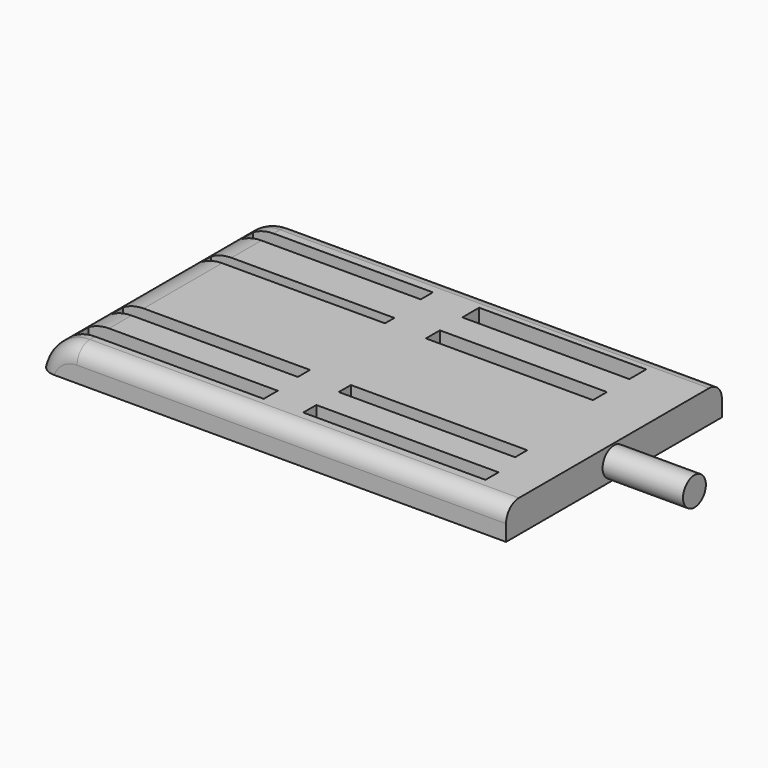
from build123d import *

# Parameters (mm, degrees)
F0_W        = 147.8525847197
F0_H        = 85.1719379425
F0_W_2      = 59.7309665754
F0_H_2      = 5.5306423455
F0_W_3      = 58.9935472235
F0_H_3      = 4.7932267189
F0_W_4      = 57.5187108479
F0_H_4      = 5.1619354635
F0_W_5      = 55.6751615368
F0_W_6      = 57.8874191269
F0_H_5      = 3.6870967597
F0_W_7      = 56.7812863737
F0_H_6      = 4.7932248563
F0_W_8      = 52.7254838962
F0_H_7      = 5.5306442082
F0_H_8      = 6.6367760301
F1_DEPTH    = 10.16
F2_T1_DEPTH = 147.3889774092
F3_R        = 5.08
F4_R        = 4.5031383634
F5_DEPTH    = 25.4


# Not quite as in the source:
# - a fillet or chamfer that OpenCascade refuses, or shapes differently, is made with other operations: its cross-section is extruded or revolved along the edge and cut away or added


with BuildPart() as f1:
    # F0 (on Top) → F1 (new body)
    with BuildSketch(Plane.XY):
        Rectangle(F0_W, F0_H)
        with Locations((-38.0981913768, -32.7256983146)):
            Rectangle(F0_W_2, F0_H_2, mode=Mode.SUBTRACT)
        with Locations((-38.4669010527, -18.7147296965)):
            Rectangle(F0_W_3, F0_H_3, mode=Mode.SUBTRACT)
        with Locations((32.6940652449, -32.5413448736)):
            Rectangle(F0_W_4, F0_H_4, mode=Mode.SUBTRACT)
        with Locations((31.7722905893, -18.7147296965)):
            Rectangle(F0_W_5, F0_H_3, mode=Mode.SUBTRACT)
        with Locations((-39.019965101, 16.4970448241)):
            Rectangle(F0_W_6, F0_H_5, mode=Mode.SUBTRACT)
        with Locations((-39.5730314776, 32.535915263)):
            Rectangle(F0_W_7, F0_H_6, mode=Mode.SUBTRACT)
        with Locations((29.1913239053, 17.4188185483)):
            Rectangle(F0_W_8, F0_H_7, mode=Mode.SUBTRACT)
        with Locations((29.1913239053, 32.3515608907)):
            Rectangle(F0_W_8, F0_H_8, mode=Mode.SUBTRACT)
    extrude(amount=F1_DEPTH)

    # F2: fillet of radius 12.7 on 1 edges, made by hand

    # F2_s2 → F2_t1 (cut)
    with BuildSketch(Plane.XZ.offset(-73.6944887046)):
        with BuildLine():
            ThreePointArc((-73.9262923598, 0), (-69.5150697233, 7.2973776994), (-61.4828844665, 10.16))
            Line((-61.4828844665, 10.16), (-73.9262923598, 10.16))
            Line((-73.9262923598, 10.16), (-73.9262923598, 0))
        make_face()
    extrude(amount=F2_T1_DEPTH, mode=Mode.SUBTRACT)

    # F3
    f3_edges = [f1.edges().sort_by_distance(p)[0] for p in [
        (6.221704, -42.585969, 10.16),
        (6.221704, 42.585969, 10.16),
        (-69.51507, 42.585969, 7.297378),
        (-69.51507, -42.585969, 7.297378),
    ]]
    fillet(f3_edges, radius=F3_R)

    # F4 (on face) → F5 (join)
    with BuildSketch(Plane.YZ.offset(73.9262923598)):
        with Locations((0, 5.0259334967)):
            Circle(F4_R)
    extrude(amount=F5_DEPTH)


solid = f1.part
